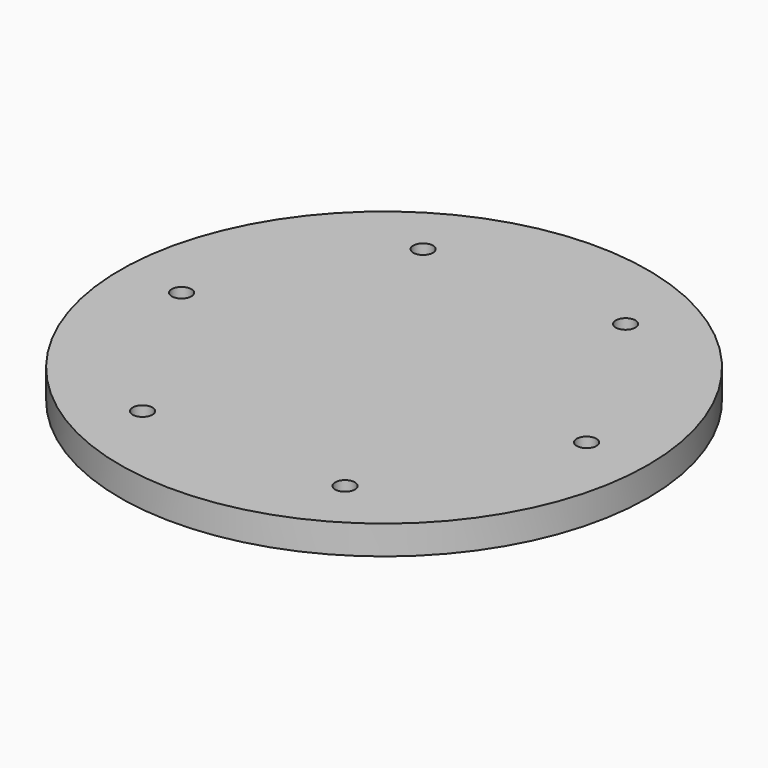
from build123d import *

# Parameters (mm, degrees)
F0_R            = 46.355
F1_DEPTH        = 5.08
F4_D            = 3.4544
F4_COPIES_COUNT = 6


# Not quite as in the source:
# - a pattern or mirror of a feature is missing from the dataset's text; its kind, count and spacing are read off the source's solid


with BuildPart() as f1:
    # F0 (on Top) → F1 (new body)
    with BuildSketch(Plane.XY):
        Circle(F0_R)
    extrude(amount=F1_DEPTH)

    # F4 (through all)
    with Locations(Plane(origin=(0, 0, 0), x_dir=(1, 0, 0), z_dir=(0, 0, -1))):
        with Locations((35.56, 0)):
            f4 = Hole(F4_D / 2)

    # F4_copies: F4 ×6 about axis
    f4_copies_axis = Axis((0, 0, 0), (0, 0, 1))
    for i in range(1, F4_COPIES_COUNT):
        add(f4.rotate(f4_copies_axis, i * 360 / F4_COPIES_COUNT), mode=Mode.SUBTRACT)


solid = f1.part
